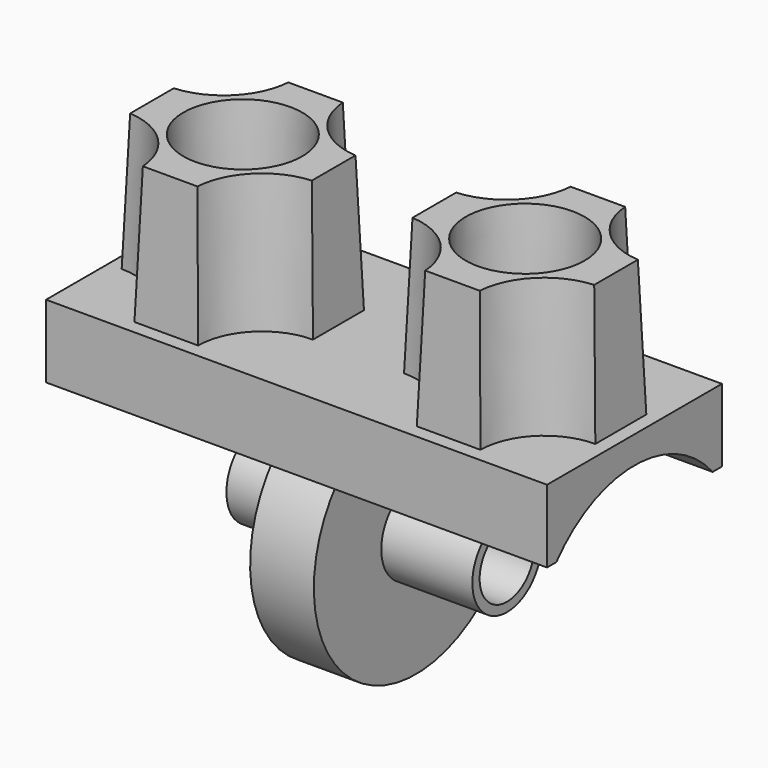
from build123d import *

# Parameters (mm, degrees)
F0_W                    = 55
F0_H                    = 24
F1_DEPTH                = 8
F3_DEPTH                = 62.03605
F4_R                    = 14
F5_DEPTH                = 3.5
F5_DEPTH_BACK           = 3.5
F7_R                    = 4.75
F7_R_2                  = 3.75
F8_DEPTH                = 10
F10_R                   = 6
F11_DEPTH               = 15
DRAFT_F11_DRAFTED_ANGLE = 2


# Not quite as in the source:
# - an extrude with a draft is written as a straight extrude whose walls are then drafted


with BuildPart() as f1:
    # F0 (on Top) → F1 (new body)
    with BuildSketch(Plane.XY):
        Rectangle(F0_W, F0_H)
    extrude(amount=F1_DEPTH)

    # F2 (on face) → F3 (cut)
    with BuildSketch(Plane(origin=(-27.5, 0, 0), x_dir=(0, -1, 0), z_dir=(-1, 0, 0))):
        with BuildLine():
            Line((-10.7238052948, 0), (10.7238052948, 0))
            ThreePointArc((10.7238052948, 0), (0, 5), (-10.7238052948, 0))
        make_face()
        with BuildLine():
            ThreePointArc((-10.7238052948, 0), (-4.7888790898, -22.1554793551), (14, -9))
            ThreePointArc((14, -9), (13.1554793551, -4.2111209102), (10.7238052948, 0))
            Line((10.7238052948, 0), (-10.7238052948, 0))
        make_face()
    extrude(amount=-F3_DEPTH, mode=Mode.SUBTRACT)

    # F4 (on Right) → F5 (join, two sides)
    with BuildSketch(Plane.YZ) as f5_sk:
        with Locations((0, -9)):
            Circle(F4_R)
    extrude(amount=F5_DEPTH)
    extrude(f5_sk.sketch, amount=-F5_DEPTH_BACK)

    # F7 (on face) → F8 (join)
    with BuildSketch(Plane.YZ.offset(3.5)):
        with Locations((0, -9)):
            Circle(F7_R)
        with Locations((0, -9)):
            Circle(F7_R_2, mode=Mode.SUBTRACT)
    extrude(amount=F8_DEPTH)

    # F9: F1 across plane


with BuildPart() as f1_1:
    add(f1.part)
    add(f1.part.mirror(Plane.YZ))


with BuildPart() as f11_drafted:
    # F10 (on face) → F11 (new body)
    with BuildSketch(Plane.XY.offset(8)):
        with BuildLine():
            Line((19, 10.5), (12, 10.5))
            ThreePointArc((12, 10.5), (9.9497474683, 5.5502525317), (5, 3.5))
            Line((5, 3.5), (5, -3.5))
            ThreePointArc((5, -3.5), (9.9497474683, -5.5502525317), (12, -10.5))
            Line((12, -10.5), (19, -10.5))
            ThreePointArc((19, -10.5), (21.0502525317, -5.5502525317), (26, -3.5))
            Line((26, -3.5), (26, 3.5))
            ThreePointArc((26, 3.5), (21.0502525317, 5.5502525317), (19, 10.5))
        make_face()
        with Locations((15.5, 0)):
            Circle(F10_R, mode=Mode.SUBTRACT)
    extrude(amount=F11_DEPTH)

    # draft_F11_drafted
    draft_f11_drafted_walls = [f11_drafted.faces().sort_by_distance(p)[0] for p in [
        (15.5, 10.5, 18),
        (9.9497474683, 5.5502525317, 18),
        (5, 0, 18),
        (9.9497474683, -5.5502525317, 18),
        (15.5, -10.5, 18),
        (21.0502525317, -5.5502525317, 18),
        (26, 0, 18),
        (21.0502525317, 5.5502525317, 18),
        (9.5, 0, 18),
    ]]
    draft(draft_f11_drafted_walls, neutral_plane=Plane.XY.offset(8), angle=DRAFT_F11_DRAFTED_ANGLE)


with BuildPart() as f1_2:
    add(f1_1.part)

    # join_F11_drafted: union F11_drafted
    add(f11_drafted.part)

    # F12: F1 across plane


with BuildPart() as f1_3:
    add(f1_2.part)
    add(f1_2.part.mirror(Plane.YZ))


solid = f1_3.part
